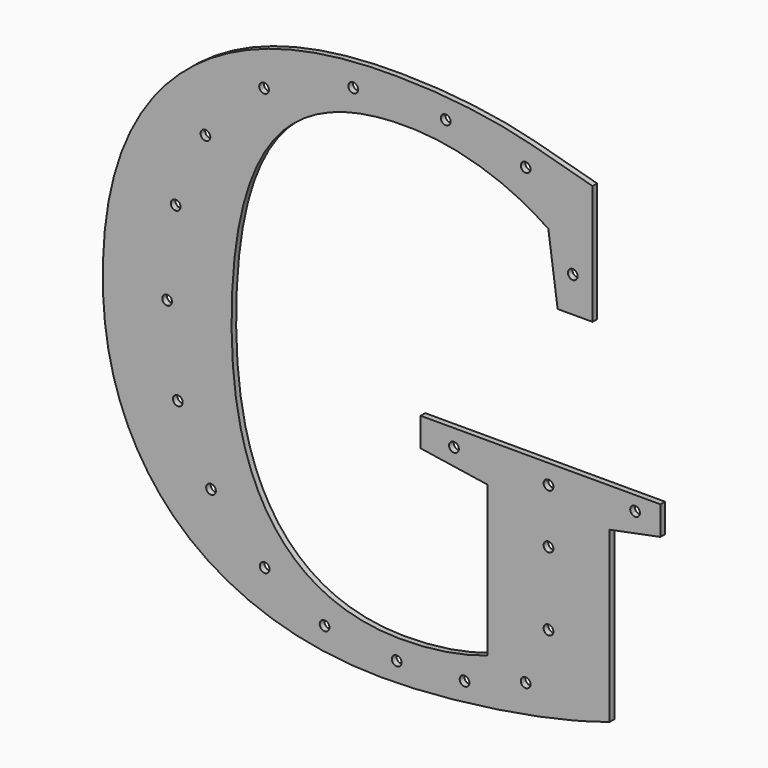
from build123d import *

# Parameters (mm, degrees)
F0_TEXT_SIZE = 1388.8888888889
F1_DEPTH     = 10
F4_DEPTH     = 12.5


# Not quite as in the source:
# - Text() gives the source's letters only with a copy of the font that has no kerning and outlines rounded to 1/6400 em; it was checked with that copy


with BuildPart() as f1:
    # F0 (on Front) → F1 (new body)
    with BuildSketch(Plane.XZ):
        with Locations((-455.5084335196, -548.7287978805)):
            Text('G', F0_TEXT_SIZE, font='Tinos', font_style=FontStyle.BOLD, text_align=(TextAlign.LEFT, TextAlign.BOTTOM))
    extrude(amount=F1_DEPTH)

    # F3 (on face) → F4 (cut, symmetric)
    with BuildSketch(Plane.XZ.offset(10)):
        with BuildLine():
            ThreePointArc((217.5483514255, -166.5712887417), (225.3765920638, -175.6937143242), (234.4990176463, -167.8654736859))
            Line((234.4990176463, -167.8654736859), (217.5483514255, -166.5712887417))
        make_face()
        with BuildLine():
            Line((217.5483514255, -166.5712887417), (234.4990176463, -167.8654736859))
            ThreePointArc((234.4990176463, -167.8654736859), (234.5175155749, -167.5421624374), (234.5236845359, -167.2183812138))
            ThreePointArc((234.5236845359, -167.2183812138), (226.3474657595, -158.7245501748), (217.5483514255, -166.5712887417))
        make_face()
        with BuildLine():
            ThreePointArc((399.6712539804, -171.6671659361), (391.1712539804, -163.1671659361), (382.6712539804, -171.6671659361))
            Line((382.6712539804, -171.6671659361), (391.1712539804, -171.6671659361))
            Line((391.1712539804, -171.6671659361), (399.6712539804, -171.6671659361))
        make_face()
        with BuildLine():
            Line((399.6712539804, -171.6671659361), (391.1712539804, -171.6671659361))
            Line((391.1712539804, -171.6671659361), (391.1712539804, -180.1671659361))
            ThreePointArc((391.1712539804, -180.1671659361), (397.1816616205, -177.6775735761), (399.6712539804, -171.6671659361))
        make_face()
        with BuildLine():
            Line((391.1712539804, -171.6671659361), (382.6712539804, -171.6671659361))
            ThreePointArc((382.6712539804, -171.6671659361), (385.1608463403, -177.6775735761), (391.1712539804, -180.1671659361))
            Line((391.1712539804, -180.1671659361), (391.1712539804, -171.6671659361))
        make_face()
        with BuildLine():
            ThreePointArc((550.9299345359, -162.7695964916), (539.7251924903, -154.7114099421), (535.651259132, -167.8979061321))
            Line((535.651259132, -167.8979061321), (550.0916685093, -166.4503345319))
            ThreePointArc((550.0916685093, -166.4503345319), (550.7177188832, -164.6570897004), (550.9299345359, -162.7695964916))
        make_face()
        with BuildLine():
            Line((550.0916685093, -166.4503345319), (535.651259132, -167.8979061321))
            ThreePointArc((535.651259132, -167.8979061321), (543.2777635244, -171.2272076204), (550.0916685093, -166.4503345319))
        make_face()
        with BuildLine():
            ThreePointArc((391.1712539804, -258.337656498), (382.6712539804, -266.837656498), (391.1712539804, -275.337656498))
            Line((391.1712539804, -275.337656498), (391.1712539804, -258.337656498))
        make_face()
        with BuildLine():
            Line((391.1712539804, -258.337656498), (391.1712539804, -275.337656498))
            ThreePointArc((391.1712539804, -275.337656498), (397.1816616205, -272.848064138), (399.6712539804, -266.837656498))
            ThreePointArc((399.6712539804, -266.837656498), (397.1816616205, -260.8272488579), (391.1712539804, -258.337656498))
        make_face()
        with BuildLine():
            ThreePointArc((391.1712539804, -385.9047961444), (382.6712539804, -394.4047961444), (391.1712539804, -402.9047961444))
            Line((391.1712539804, -402.9047961444), (391.1712539804, -385.9047961444))
        make_face()
        with BuildLine():
            Line((391.1712539804, -385.9047961444), (391.1712539804, -402.9047961444))
            ThreePointArc((391.1712539804, -402.9047961444), (397.1816616205, -400.4152037845), (399.6712539804, -394.4047961444))
            ThreePointArc((399.6712539804, -394.4047961444), (397.1816616205, -388.3943885043), (391.1712539804, -385.9047961444))
        make_face()
        with BuildLine():
            ThreePointArc((359.7092989539, -488.4801204658), (359.501722918, -486.6131162346), (358.8891331188, -484.8372991416))
            add(Edge.make_bspline(
                [(343.4805224969, -492.0179184359), (348.6682655393, -489.6909583865), (353.798342016, -487.2895035632), (358.8891331188, -484.8372991416)],
                knots=[0.9376471171, 0.9376471171, 0.9376471171, 0.9376471171, 0.9575220704, 0.9575220704, 0.9575220704, 0.9575220704], degree=3))
            ThreePointArc((343.4805224969, -492.0179184359), (353.0197409048, -496.7850768138), (359.7092989539, -488.4801204658))
        make_face()
        with BuildLine():
            add(Edge.make_bspline(
                [(343.4805224969, -492.0179184359), (348.6682655393, -489.6909583865), (353.798342016, -487.2895035632), (358.8891331188, -484.8372991416)],
                knots=[0.9376471171, 0.9376471171, 0.9376471171, 0.9376471171, 0.9575220704, 0.9575220704, 0.9575220704, 0.9575220704], degree=3))
            ThreePointArc((358.8891331188, -484.8372991416), (347.6189059114, -480.7756362001), (343.4805224969, -492.0179184359))
        make_face()
        with BuildLine():
            add(Edge.make_bspline(
                [(236.0622794556, -521.8438218801), (241.7310744628, -521.1560881261), (247.3494336936, -520.3817416925), (252.9000711644, -519.5059376337)],
                knots=[0.813809332, 0.813809332, 0.813809332, 0.813809332, 0.8315791974, 0.8315791974, 0.8315791974, 0.8315791974], degree=3))
            ThreePointArc((236.0622794556, -521.8438218801), (245.0396210668, -529.2324148501), (252.9916192128, -520.7500983052))
            ThreePointArc((252.9916192128, -520.7500983052), (252.9687013048, -520.1263361667), (252.9000711644, -519.5059376337))
        make_face()
        with BuildLine():
            ThreePointArc((252.9000711644, -519.5059376337), (243.322630435, -512.3308664378), (236.0622794556, -521.8438218801))
            add(Edge.make_bspline(
                [(236.0622794556, -521.8438218801), (241.7310744628, -521.1560881261), (247.3494336936, -520.3817416925), (252.9000711644, -519.5059376337)],
                knots=[0.813809332, 0.813809332, 0.813809332, 0.813809332, 0.8315791974, 0.8315791974, 0.8315791974, 0.8315791974], degree=3))
        make_face()
        with BuildLine():
            add(Edge.make_bspline(
                [(117.5531294054, -528.4815006618), (123.1814881405, -528.3523981419), (128.8419426635, -528.1829713677), (134.5463374808, -528.0024233864)],
                knots=[0.6916453035, 0.6916453035, 0.6916453035, 0.6916453035, 0.7095309121, 0.7095309121, 0.7095309121, 0.7095309121], degree=3))
            ThreePointArc((134.5463374808, -528.0024233864), (125.8107146886, -519.7637986112), (117.5531294054, -528.4815006618))
        make_face()
        with BuildLine():
            ThreePointArc((134.5502538917, -528.2604227038), (134.5492747326, -528.1314081832), (134.5463374808, -528.0024233864))
            add(Edge.make_bspline(
                [(117.5531294054, -528.4815006618), (123.1814881405, -528.3523981419), (128.8419426635, -528.1829713677), (134.5463374808, -528.0024233864)],
                knots=[0.6916453035, 0.6916453035, 0.6916453035, 0.6916453035, 0.7095309121, 0.7095309121, 0.7095309121, 0.7095309121], degree=3))
            ThreePointArc((117.5531294054, -528.4815006618), (126.1608022207, -536.759703795), (134.5502538917, -528.2604227038))
        make_face()
        with BuildLine():
            ThreePointArc((8.5, -515.2441263199), (1.3950206156, -506.8593831824), (-8.0420982311, -512.4919170179))
            add(Edge.make_bspline(
                [(-8.0420982311, -512.4919170179), (-5.3521021137, -513.4603243141), (0.0610603521, -515.3139191346), (5.429691649, -516.9530554114), (8.1287758498, -517.7286792339)],
                knots=[0.5581392707, 0.5581392707, 0.5581392707, 0.5581392707, 0.5664325749, 0.5748809283, 0.5748809283, 0.5748809283, 0.5748809283], degree=3))
            ThreePointArc((8.1287758499, -517.728679234), (8.4066817093, -516.500192655), (8.5, -515.2441263199))
        make_face()
        with BuildLine():
            add(Edge.make_bspline(
                [(-8.0420982311, -512.4919170179), (-5.3521021137, -513.4603243141), (0.0610603521, -515.3139191346), (5.429691649, -516.9530554114), (8.1287758498, -517.7286792339)],
                knots=[0.5581392707, 0.5581392707, 0.5581392707, 0.5581392707, 0.5664325749, 0.5748809283, 0.5748809283, 0.5748809283, 0.5748809283], degree=3))
            ThreePointArc((-8.0420982311, -512.4919170179), (-2.6187397502, -523.3306708304), (8.1287758499, -517.728679234))
        make_face()
        with BuildLine():
            ThreePointArc((-96.2371467911, -459.849494169), (-102.0969624727, -451.7699256926), (-111.5970119122, -454.8303059359))
            add(Edge.make_bspline(
                [(-111.5970119122, -454.8303059359), (-107.0672377056, -458.2036062924), (-102.4611333564, -461.5156012997), (-97.7932707861, -464.751798324)],
                knots=[0.4506367838, 0.4506367838, 0.4506367838, 0.4506367838, 0.4656705, 0.4656705, 0.4656705, 0.4656705], degree=3))
            ThreePointArc((-97.7932707861, -464.751798324), (-96.6355128188, -462.4211720219), (-96.2371467911, -459.849494169))
        make_face()
        with BuildLine():
            add(Edge.make_bspline(
                [(-111.5970119122, -454.8303059359), (-107.0672377056, -458.2036062924), (-102.4611333564, -461.5156012997), (-97.7932707861, -464.751798324)],
                knots=[0.4506367838, 0.4506367838, 0.4506367838, 0.4506367838, 0.4656705, 0.4656705, 0.4656705, 0.4656705], degree=3))
            ThreePointArc((-111.5970119122, -454.8303059359), (-109.6980708238, -466.7516121585), (-97.7932707861, -464.751798324))
        make_face()
        with BuildLine():
            add(Edge.make_bspline(
                [(-203.4496977516, -362.9765634604), (-200.213395616, -367.580486895), (-196.8424043864, -372.1281288175), (-193.3243153987, -376.6305136707)],
                knots=[0.3240958487, 0.3240958487, 0.3240958487, 0.3240958487, 0.3420406222, 0.3420406222, 0.3420406222, 0.3420406222], degree=3))
            ThreePointArc((-193.3243153987, -376.6305136707), (-190.8570632101, -373.641382543), (-189.9734021359, -369.8676070639))
            ThreePointArc((-189.9734021359, -369.8676070639), (-194.6035515402, -362.2996313526), (-203.4496977516, -362.9765634604))
        make_face()
        with BuildLine():
            ThreePointArc((-203.4496977516, -362.9765634604), (-205.3009238883, -374.9307036184), (-193.3243153987, -376.6305136707))
            add(Edge.make_bspline(
                [(-203.4496977516, -362.9765634604), (-200.213395616, -367.580486895), (-196.8424043864, -372.1281288175), (-193.3243153987, -376.6305136707)],
                knots=[0.3240958487, 0.3240958487, 0.3240958487, 0.3240958487, 0.3420406222, 0.3420406222, 0.3420406222, 0.3420406222], degree=3))
        make_face()
        with BuildLine():
            add(Edge.make_bspline(
                [(-258.8890753168, -244.3157278347), (-257.2612682292, -249.7087508102), (-255.5356551998, -255.1177132446), (-253.7186954465, -260.5098271213)],
                knots=[0.1868912991, 0.1868912991, 0.1868912991, 0.1868912991, 0.2042190503, 0.2042190503, 0.2042190503, 0.2042190503], degree=3))
            ThreePointArc((-253.7186954465, -260.5098271213), (-249.4846024488, -257.4197371353), (-247.8683554116, -252.4333611819))
            ThreePointArc((-247.8683554116, -252.4333611819), (-251.3273296823, -245.5895274904), (-258.8890753168, -244.3157278348))
        make_face()
        with BuildLine():
            ThreePointArc((-258.8890753168, -244.3157278348), (-264.4656617112, -255.0186330612), (-253.7186954465, -260.5098271213))
            add(Edge.make_bspline(
                [(-258.8890753168, -244.3157278347), (-257.2612682292, -249.7087508102), (-255.5356551998, -255.1177132446), (-253.7186954465, -260.5098271213)],
                knots=[0.1868912991, 0.1868912991, 0.1868912991, 0.1868912991, 0.2042190503, 0.2042190503, 0.2042190503, 0.2042190503], degree=3))
        make_face()
        with BuildLine():
            ThreePointArc((-266.5613849085, -103.8503256583), (-266.5614204769, -103.825735803), (-266.5615271817, -103.8011461536))
            Line((-266.5615271817, -103.8011461536), (-275.0613849085, -103.8503256583))
            add(Edge.make_bspline(
                [(-275.0613849085, -103.8503256583), (-275.2713359357, -106.6704003117), (-275.481286963, -109.4904749651), (-275.6785823025, -112.3278882429)],
                knots=[0, 0, 0, 0, 0.0143786991, 0.0143786991, 0.0143786991, 0.0143786991], degree=3))
            ThreePointArc((-275.6785823025, -112.3278882429), (-269.2733013677, -110.0751219541), (-266.5613849085, -103.8503256583))
        make_face()
        with BuildLine():
            add(Edge.make_bspline(
                [(-275.0613849085, -103.8503256583), (-275.2713359357, -106.6704003117), (-275.481286963, -109.4904749651), (-275.6785823025, -112.3278882429)],
                knots=[0, 0, 0, 0, 0.0143786991, 0.0143786991, 0.0143786991, 0.0143786991], degree=3))
            Line((-275.0613849085, -103.8503256583), (-283.5612426353, -103.899505163))
            ThreePointArc((-283.5612426353, -103.899505163), (-281.26941067, -109.6563928423), (-275.6785823025, -112.3278882429))
        make_face()
        with BuildLine():
            Line((-283.5612426353, -103.899505163), (-275.0613849085, -103.8503256583))
            add(Edge.make_bspline(
                [(-275.0613849085, -103.8503256583), (-275.1462276283, -101.0182754674), (-275.2310703481, -98.1862252766), (-275.3120007825, -95.3540210684)],
                knots=[0, 0, 0, 0, 0.0102934651, 0.0102934651, 0.0102934651, 0.0102934651], degree=3))
            ThreePointArc((-275.3120007825, -95.3540210684), (-281.1768588609, -97.9468539392), (-283.5612426353, -103.899505163))
        make_face()
        with BuildLine():
            Line((-275.0613849085, -103.8503256583), (-266.5615271817, -103.8011461536))
            ThreePointArc((-266.5615271817, -103.8011461536), (-269.1579131895, -97.7348517059), (-275.3120007825, -95.3540210684))
            add(Edge.make_bspline(
                [(-275.0613849085, -103.8503256583), (-275.1462276283, -101.0182754674), (-275.2310703481, -98.1862252766), (-275.3120007825, -95.3540210684)],
                knots=[0, 0, 0, 0, 0.0102934651, 0.0102934651, 0.0102934651, 0.0102934651], degree=3))
        make_face()
        with BuildLine():
            add(Edge.make_bspline(
                [(-262.5650229709, 38.8832637646), (-261.8285712965, 41.5634677529), (-260.3064618162, 46.9109087352), (-258.6274760532, 52.4416740484), (-257.7685233827, 55.1919103176)],
                knots=[0.166644604, 0.166644604, 0.166644604, 0.166644604, 0.1746869609, 0.1824344167, 0.1824344167, 0.1824344167, 0.1824344167], degree=3))
            ThreePointArc((-262.5650229709, 38.8832637646), (-255.1155853791, 40.2747077316), (-251.7373361588, 47.058340162))
            ThreePointArc((-251.7373361588, 47.058340162), (-253.4096385748, 52.1211996013), (-257.7685233826, 55.1919103177))
        make_face()
        with BuildLine():
            ThreePointArc((-257.7685233826, 55.1919103177), (-268.391964736, 49.4566797475), (-262.5650229709, 38.8832637646))
            add(Edge.make_bspline(
                [(-262.5650229709, 38.8832637646), (-261.8285712965, 41.5634677529), (-260.3064618162, 46.9109087352), (-258.6274760532, 52.4416740484), (-257.7685233827, 55.1919103176)],
                knots=[0.166644604, 0.166644604, 0.166644604, 0.166644604, 0.1746869609, 0.1824344167, 0.1824344167, 0.1824344167, 0.1824344167], degree=3))
        make_face()
        with BuildLine():
            ThreePointArc((-199.6707566977, 171.3463068008), (-200.768975807, 175.5252587804), (-203.7798483793, 178.6243507785))
            add(Edge.make_bspline(
                [(-212.3603489535, 163.9505433696), (-210.9639569093, 166.4878196494), (-208.0994287634, 171.546862448), (-205.242875065, 176.2784828177), (-203.7798483794, 178.6243507785)],
                knots=[0.2828980715, 0.2828980715, 0.2828980715, 0.2828980715, 0.291043404, 0.2995933941, 0.2995933941, 0.2995933941, 0.2995933941], degree=3))
            ThreePointArc((-212.3603489534, 163.9505433696), (-203.8906593959, 164.0025497864), (-199.6707566977, 171.3463068008))
        make_face()
        with BuildLine():
            add(Edge.make_bspline(
                [(-212.3603489535, 163.9505433696), (-210.9639569093, 166.4878196494), (-208.0994287634, 171.546862448), (-205.242875065, 176.2784828177), (-203.7798483794, 178.6243507785)],
                knots=[0.2828980715, 0.2828980715, 0.2828980715, 0.2828980715, 0.291043404, 0.2995933941, 0.2995933941, 0.2995933941, 0.2995933941], degree=3))
            ThreePointArc((-203.7798483793, 178.6243507785), (-215.5083508543, 175.6369608294), (-212.3603489534, 163.9505433696))
        make_face()
        with BuildLine():
            ThreePointArc((-98.5306353352, 281.6981417662), (-110.3752399786, 284.2690235844), (-112.7487035051, 272.3832857709))
            add(Edge.make_bspline(
                [(-112.7487035051, 272.3832857709), (-110.4350276408, 274.0093501263), (-105.758171522, 277.1889182781), (-100.9599144114, 280.2208984999), (-98.5306353352, 281.6981417662)],
                knots=[0.4538494931, 0.4538494931, 0.4538494931, 0.4538494931, 0.4635415693, 0.473190152, 0.473190152, 0.473190152, 0.473190152], degree=3))
        make_face()
        with BuildLine():
            add(Edge.make_bspline(
                [(-112.7487035051, 272.3832857709), (-110.4350276408, 274.0093501263), (-105.758171522, 277.1889182781), (-100.9599144114, 280.2208984999), (-98.5306353352, 281.6981417662)],
                knots=[0.4538494931, 0.4538494931, 0.4538494931, 0.4538494931, 0.4635415693, 0.473190152, 0.473190152, 0.473190152, 0.473190152], degree=3))
            ThreePointArc((-112.7487035051, 272.3832857709), (-103.2189737207, 269.0344113183), (-97.2171672583, 277.1590054035))
            ThreePointArc((-97.2171672583, 277.1590054035), (-97.5521344553, 279.5216817095), (-98.5306353352, 281.6981417662))
        make_face()
        with BuildLine():
            add(Edge.make_bspline(
                [(41.5637537256, 327.1567165351), (47.1316096393, 328.0573923098), (52.7449630313, 328.8987406039), (58.3756991871, 329.6764072186)],
                knots=[0.61185812, 0.61185812, 0.61185812, 0.61185812, 0.6250117883, 0.6250117883, 0.6250117883, 0.6250117883], degree=3))
            ThreePointArc((58.375699187, 329.6764072186), (48.7025804564, 336.8712462484), (41.5637537256, 327.1567165351))
        make_face()
        with BuildLine():
            ThreePointArc((58.4624468295, 328.4651331917), (58.4407321821, 329.0723213672), (58.375699187, 329.6764072186))
            add(Edge.make_bspline(
                [(41.5637537256, 327.1567165351), (47.1316096393, 328.0573923098), (52.7449630313, 328.8987406039), (58.3756991871, 329.6764072186)],
                knots=[0.61185812, 0.61185812, 0.61185812, 0.61185812, 0.6250117883, 0.6250117883, 0.6250117883, 0.6250117883], degree=3))
            ThreePointArc((41.5637537256, 327.1567165351), (50.6186132022, 319.9904977605), (58.4624468295, 328.4651331917))
        make_face()
        with BuildLine():
            add(Edge.make_bspline(
                [(203.0559133829, 332.6175910129), (208.6819867073, 332.0041588088), (214.2953324555, 331.3260871363), (219.9353943735, 330.5986495319)],
                knots=[0.7478315112, 0.7478315112, 0.7478315112, 0.7478315112, 0.7638386751, 0.7638386751, 0.7638386751, 0.7638386751], degree=3))
            ThreePointArc((219.9353943734, 330.5986495319), (219.9842986247, 331.1231375569), (220.0006209373, 331.6496476673))
            ThreePointArc((220.0006209373, 331.6496476673), (211.9853815934, 340.1358132977), (203.0559133829, 332.6175910129))
        make_face()
        with BuildLine():
            ThreePointArc((203.0559133829, 332.6175910129), (210.4911379768, 323.2098050057), (219.9353943734, 330.5986495319))
            add(Edge.make_bspline(
                [(203.0559133829, 332.6175910129), (208.6819867073, 332.0041588088), (214.2953324555, 331.3260871363), (219.9353943735, 330.5986495319)],
                knots=[0.7478315112, 0.7478315112, 0.7478315112, 0.7478315112, 0.7638386751, 0.7638386751, 0.7638386751, 0.7638386751], degree=3))
        make_face()
        with BuildLine():
            add(Edge.make_bspline(
                [(343.2617784569, 306.9617439382), (348.7245647259, 305.0269006384), (353.9899907, 302.8988442837), (358.9977978069, 300.5429884368)],
                knots=[0.8759628467, 0.8759628467, 0.8759628467, 0.8759628467, 0.8920501951, 0.8920501951, 0.8920501951, 0.8920501951], degree=3))
            ThreePointArc((358.9977978069, 300.5429884368), (359.5295225161, 302.2083617511), (359.7092989539, 303.947292421))
            ThreePointArc((359.7092989539, 303.947292421), (352.7416298215, 312.3080317491), (343.2617784569, 306.9617439382))
        make_face()
        with BuildLine():
            ThreePointArc((343.2617784569, 306.9617439382), (347.9989364327, 296.0768685136), (358.9977978069, 300.5429884368))
            add(Edge.make_bspline(
                [(343.2617784569, 306.9617439382), (348.7245647259, 305.0269006384), (353.9899907, 302.8988442837), (358.9977978069, 300.5429884368)],
                knots=[0.8759628467, 0.8759628467, 0.8759628467, 0.8759628467, 0.8920501951, 0.8920501951, 0.8920501951, 0.8920501951], degree=3))
        make_face()
        with BuildLine():
            ThreePointArc((442.0432157859, 165.9565798513), (439.3524687636, 172.1616245604), (432.983785235, 174.4381503108))
            Line((432.983785235, 174.4381503108), (434.1026463369, 157.4750093919))
            ThreePointArc((434.1026463369, 157.4750093919), (439.748260495, 160.1473268737), (442.0432157859, 165.9565798513))
        make_face()
        with BuildLine():
            Line((434.1026463369, 157.4750093919), (432.983785235, 174.4381503108))
            ThreePointArc((432.983785235, 174.4381503108), (425.0616453265, 165.3971493004), (434.1026463369, 157.4750093919))
        make_face()
    extrude(amount=F4_DEPTH, both=True, mode=Mode.SUBTRACT)


solid = f1.part
